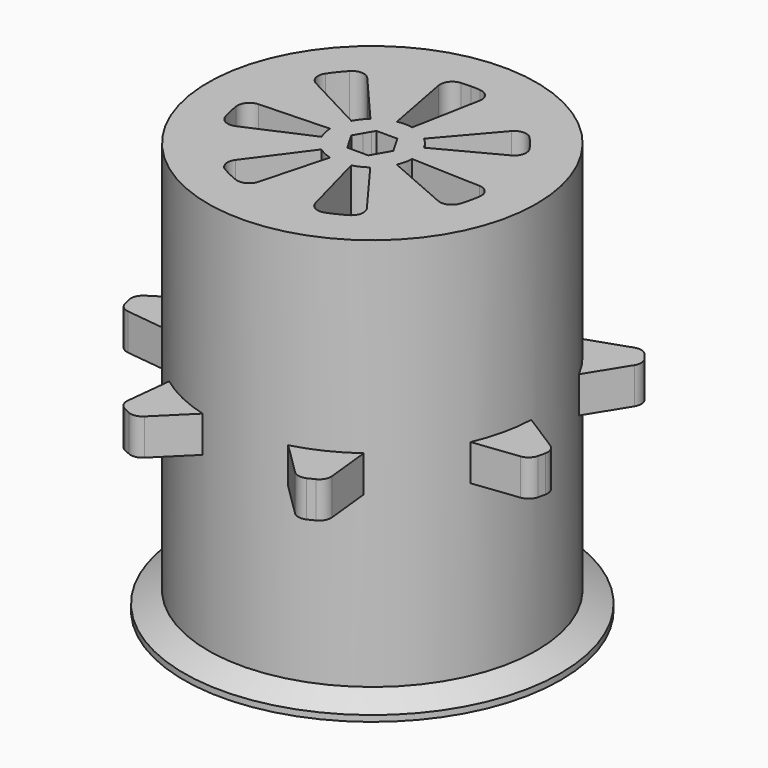
from build123d import *

# Parameters (mm, degrees)
F0_R     = 13.57391
F1_DEPTH = 17
F3_DEPTH = 1.5
F5_DEPTH = 34
F6_R     = 1
F7_R     = 15.57391
F7_R_2   = 13.57391
F8_DEPTH = 1.5
F9_SIZE2 = 0.99999
F9_SIZE  = 1.99999
F10_R    = 1


# Not quite as in the source:
# - a fillet or chamfer is up to 0.001 mm smaller than in the source, because OpenCascade refuses the exact size
# - a feature names something its author has since deleted; it is built from what else it names


with BuildPart() as f1:
    # F0 (on Top) → F1 (new body, symmetric)
    with BuildSketch(Plane.XY):
        Circle(F0_R)
    extrude(amount=F1_DEPTH, both=True)

    # F2 (on Top) → F3 (join, symmetric)
    with BuildSketch(Plane.XY):
        with BuildLine():
            Line((-8.8722387473, 10.27299432), (-13.094084175, 11.721231689))
            ThreePointArc((-13.094084175, 11.721231689), (-13.7398361081, 10.9571536638), (-14.3410637787, 10.1575687241))
            Line((-14.3410637787, 10.1575687241), (-11.9896877566, 6.3638369077))
            ThreePointArc((-11.9896877566, 6.3638369077), (-10.6125101782, 8.4631944563), (-8.8722387473, 10.27299432))
        make_face()
        with BuildLine():
            ThreePointArc((1, 17.5454356654), (0, 17.57391), (-1, 17.5454356654))
            Line((-1, 17.5454356654), (-2.5, 13.3417027657))
            ThreePointArc((-2.5, 13.3417027657), (0, 13.57391), (2.5, 13.3417027657))
            Line((2.5, 13.3417027657), (1, 17.5454356654))
        make_face()
        with BuildLine():
            Line((11.9896877566, 6.3638369077), (14.3410637787, 10.1575687241))
            ThreePointArc((14.3410637787, 10.1575687241), (13.7398361081, 10.9571536638), (13.094084175, 11.721231689))
            Line((13.094084175, 11.721231689), (8.8722387473, 10.27299432))
            ThreePointArc((8.8722387473, 10.27299432), (10.6125101782, 8.4631944563), (11.9896877566, 6.3638369077))
        make_face()
        with BuildLine():
            Line((12.4508960874, -5.4061279404), (16.8830140276, -4.8791546431))
            ThreePointArc((16.8830140276, -4.8791546431), (17.1332953852, -3.9105628665), (17.3280558955, -2.9292988187))
            Line((17.3280558955, -2.9292988187), (13.5635007572, -0.5314883795))
            ThreePointArc((13.5635007572, -0.5314883795), (13.2335837364, -3.0204791306), (12.4508960874, -5.4061279404))
        make_face()
        with BuildLine():
            Line((3.5363257124, -13.1051681845), (6.711710363, -16.2417750474))
            ThreePointArc((6.711710363, -16.2417750474), (7.6250337817, -15.8335457973), (8.5136480988, -15.3740075692))
            Line((8.5136480988, -15.3740075692), (8.0411700519, -10.9357494889))
            ThreePointArc((8.0411700519, -10.9357494889), (5.8894988252, -12.2296703257), (3.5363257124, -13.1051681845))
        make_face()
        with BuildLine():
            Line((-8.0411700519, -10.9357494889), (-8.5136480988, -15.3740075692))
            ThreePointArc((-8.5136480988, -15.3740075692), (-7.6250337817, -15.8335457973), (-6.711710363, -16.2417750474))
            Line((-6.711710363, -16.2417750474), (-3.5363257124, -13.1051681845))
            ThreePointArc((-3.5363257124, -13.1051681845), (-5.8894988252, -12.2296703257), (-8.0411700519, -10.9357494889))
        make_face()
        with BuildLine():
            Line((-13.5635007572, -0.5314883795), (-17.3280558955, -2.9292988187))
            ThreePointArc((-17.3280558955, -2.9292988187), (-17.1332953852, -3.9105628665), (-16.8830140276, -4.8791546431))
            Line((-16.8830140276, -4.8791546431), (-12.4508960874, -5.4061279404))
            ThreePointArc((-12.4508960874, -5.4061279404), (-13.2335837364, -3.0204791306), (-13.5635007572, -0.5314883795))
        make_face()
    extrude(amount=F3_DEPTH, both=True)

    # F4 (on face) → F5 (cut)
    with BuildSketch(Plane.XY.offset(17)):
        with BuildLine():
            ThreePointArc((-3.0007085232, 1.5847516846), (-2.6531275445, 2.1157986141), (-2.2127391143, 2.5728340707))
            Line((-2.2127391143, 2.5728340707), (-6.6382173429, 7.718502212))
            ThreePointArc((-6.6382173429, 7.718502212), (-7.9593826336, 6.3473958423), (-9.0021255696, 4.7542550537))
            Line((-9.0021255696, 4.7542550537), (-3.0007085232, 1.5847516846))
        make_face()
        with BuildLine():
            ThreePointArc((-0.6319024037, 3.334124907), (-0.3173418417, 3.3786067688), (0, 3.3934775))
            Line((0, 3.3934775), (0, 6.786955))
            Line((0, 6.786955), (0, 10.1804325))
            ThreePointArc((0, 10.1804325), (-0.9520255252, 10.1358203065), (-1.895707211, 10.0023747209))
            Line((-1.895707211, 10.0023747209), (-0.6319024037, 3.334124907))
        make_face()
        with BuildLine():
            Line((0, 6.786955), (0, 3.3934775))
            ThreePointArc((0, 3.3934775), (0.3173418417, 3.3786067688), (0.6319024037, 3.334124907))
            Line((0.6319024037, 3.334124907), (1.895707211, 10.0023747209))
            ThreePointArc((1.895707211, 10.0023747209), (0.9520255252, 10.1358203065), (0, 10.1804325))
            Line((0, 10.1804325), (0, 6.786955))
        make_face()
        with BuildLine():
            ThreePointArc((2.2127391143, 2.5728340707), (2.6531275445, 2.1157986141), (3.0007085232, 1.5847516846))
            Line((3.0007085232, 1.5847516846), (9.0021255696, 4.7542550537))
            ThreePointArc((9.0021255696, 4.7542550537), (7.9593826336, 6.3473958423), (6.6382173429, 7.718502212))
            Line((6.6382173429, 7.718502212), (2.2127391143, 2.5728340707))
        make_face()
        with BuildLine():
            ThreePointArc((3.3911429475, -0.1258532971), (3.3083959341, -0.7551197827), (3.1099199215, -1.3579718793))
            Line((3.1099199215, -1.3579718793), (9.3297597644, -4.073915638))
            ThreePointArc((9.3297597644, -4.073915638), (9.9251878023, -2.265359348), (10.1734288426, -0.3775598913))
            Line((10.1734288426, -0.3775598913), (3.3911429475, -0.1258532971))
        make_face()
        with BuildLine():
            ThreePointArc((2.0159469746, -2.7297705652), (1.4723747063, -3.0574175814), (0.8772981881, -3.2781149205))
            Line((0.8772981881, -3.2781149205), (2.6318945642, -9.8343447616))
            ThreePointArc((2.6318945642, -9.8343447616), (4.4171241189, -9.1722527443), (6.0478409237, -8.1893116956))
            Line((6.0478409237, -8.1893116956), (2.0159469746, -2.7297705652))
        make_face()
        with BuildLine():
            ThreePointArc((-0.8772981881, -3.2781149205), (-1.4723747063, -3.0574175814), (-2.0159469746, -2.7297705652))
            Line((-2.0159469746, -2.7297705652), (-6.0478409237, -8.1893116956))
            ThreePointArc((-6.0478409237, -8.1893116956), (-4.4171241189, -9.1722527443), (-2.6318945642, -9.8343447616))
            Line((-2.6318945642, -9.8343447616), (-0.8772981881, -3.2781149205))
        make_face()
        with BuildLine():
            ThreePointArc((-3.1099199215, -1.3579718793), (-3.3083959341, -0.7551197827), (-3.3911429475, -0.1258532971))
            Line((-3.3911429475, -0.1258532971), (-10.1734288426, -0.3775598913))
            ThreePointArc((-10.1734288426, -0.3775598913), (-9.9251878023, -2.265359348), (-9.3297597644, -4.073915638))
            Line((-9.3297597644, -4.073915638), (-3.1099199215, -1.3579718793))
        make_face()
        Polygon((1.3273298856, 0.7009971998), (0, 0), (1.6957169725, -0.0629320484), (1.7320508076, 0), align=None)
        Polygon((1.6957169725, -0.0629320484), (0, 0), (1.3833114811, -0.6040342321), align=None)
        Polygon((1.3833114811, -0.6040342321), (0, 0), (0.9720883359, -1.3162936127), align=None)
        Polygon((0.9720883359, -1.3162936127), (0, 0), (0.4014341516, -1.5), (0.8660254038, -1.5), align=None)
        Polygon((0.4014341516, -1.5), (0, 0), (-0.4014341516, -1.5), align=None)
        Polygon((-0.4014341516, -1.5), (0, 0), (-0.9720883359, -1.3162936127), (-0.8660254038, -1.5), align=None)
        Polygon((-0.9720883359, -1.3162936127), (0, 0), (-1.3833114811, -0.6040342321), align=None)
        Polygon((-1.3833114811, -0.6040342321), (0, 0), (-1.6957169725, -0.0629320484), align=None)
        Polygon((-1.6957169725, -0.0629320484), (0, 0), (-1.3273298856, 0.7009971998), (-1.7320508076, 0), align=None)
        Polygon((-1.3273298856, 0.7009971998), (0, 0), (-1.0363453205, 1.2049972508), align=None)
        Polygon((-1.0363453205, 1.2049972508), (0, 0), (-0.2842885711, 1.5), (-0.8660254038, 1.5), align=None)
        Polygon((-0.2842885711, 1.5), (0, 0), (0, 1.5), align=None)
        Polygon((0, 1.5), (0, 0), (0.2842885711, 1.5), align=None)
        Polygon((0.2842885711, 1.5), (0, 0), (1.0363453205, 1.2049972508), (0.8660254038, 1.5), align=None)
        Polygon((1.0363453205, 1.2049972508), (0, 0), (1.3273298856, 0.7009971998), align=None)
    extrude(amount=-F5_DEPTH, mode=Mode.SUBTRACT)

    # F6
    f6_edges = [f1.edges().sort_by_distance(p)[0] for p in [
        (-6.047841, -8.189312, 0),
        (-2.631895, -9.834345, 0),
        (2.631895, -9.834345, 0),
        (6.047841, -8.189312, 0),
        (9.32976, -4.073916, 0),
        (-9.32976, -4.073916, 0),
        (-10.173429, -0.37756, 0),
        (-9.002126, 4.754255, 0),
        (-6.638217, 7.718502, 0),
        (6.638217, 7.718502, 0),
        (-1.895707, 10.002375, 0),
        (1.895707, 10.002375, 0),
        (9.002126, 4.754255, 0),
        (10.173429, -0.37756, 0),
    ]]
    fillet(f6_edges, radius=F6_R)

    # F7 (on face) → F8 (join)
    with BuildSketch(Plane(origin=(0, 0, -17), x_dir=(1, 0, 0), z_dir=(0, 0, -1))):
        Circle(F7_R)
        Circle(F7_R_2, mode=Mode.SUBTRACT)
    extrude(amount=-F8_DEPTH)

    # F9 (size 2 and 1 in the source; OpenCascade refuses exactly that, so slightly less here)
    f9_edges = [f1.edges().sort_by_distance(p)[0] for p in [
        (-15.57391, 0, -15.5),
    ]]
    f9_side = f1.faces().sort_by_distance((-15.133413, 0, -15.5))[0]
    chamfer(f9_edges, length=F9_SIZE, length2=F9_SIZE2, reference=f9_side)

    # F10
    f10_edges = [f1.edges().sort_by_distance(p)[0] for p in [
        (14.341064, 10.157569, 0),
        (13.094084, 11.721232, 0),
        (1, 17.545436, 0),
        (-1, 17.545436, 0),
        (-13.094084, 11.721232, 0),
        (-14.341064, 10.157569, 0),
        (-17.328056, -2.929299, 0),
        (-16.883014, -4.879155, 0),
        (-8.513648, -15.374008, 0),
        (-6.71171, -16.241775, 0),
        (6.71171, -16.241775, 0),
        (8.513648, -15.374008, 0),
        (16.883014, -4.879155, 0),
        (17.328056, -2.929299, 0),
    ]]
    fillet(f10_edges, radius=F10_R)


solid = f1.part
